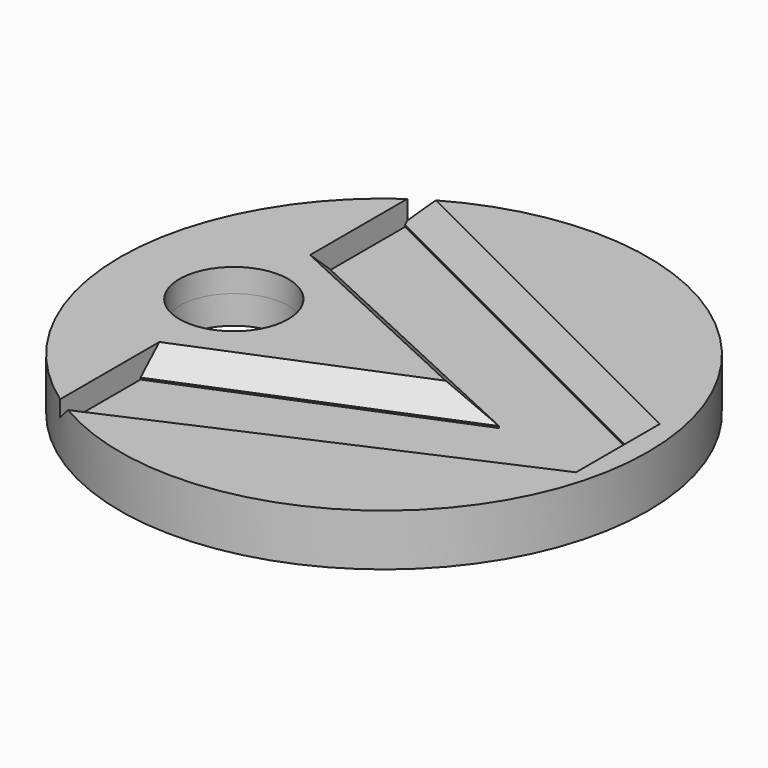
from build123d import *

# Parameters (mm, degrees)
F0_R         = 12.125
F0_R_2       = 2.5
F1_DEPTH     = 2.38
F2_R         = 12.125
F3_DEPTH     = 1.3
F4_T4_DEPTH  = 25.2617303144
F4_T10_DEPTH = 18.811479046
F4_T15_DEPTH = 18.5490461255
F4_T20_DEPTH = 24.8150280867
F5_R         = 2.5
F6_DEPTH     = 25


# Not quite as in the source:
# - a fillet or chamfer that OpenCascade refuses, or shapes differently, is made with other operations: its cross-section is extruded or revolved along the edge and cut away or added


with BuildPart() as f1:
    # F0 (on Top) → F1 (new body)
    with BuildSketch(Plane.XY):
        Circle(F0_R)
        with Locations((-6.9000022486, 0)):
            Circle(F0_R_2, mode=Mode.SUBTRACT)
        Polygon((-6.9049564988, -9.6863286317), (-6.9049564988, -5.3536104666), (5.4957817031, -0.2610715792), (-6.9049564988, 5.4868851832), (-6.9049564988, 9.8370038228), (11.0929343528, 0.8467586343), (11.0929343528, -1.7459120749), align=None, mode=Mode.SUBTRACT)
    extrude(amount=F1_DEPTH)

    # F2 (on Top) → F3 (join)
    with BuildSketch(Plane.XY):
        Circle(F2_R)
    extrude(amount=F3_DEPTH)

    # F4: chamfer of 1 on 4 edges, made by hand


with BuildPart() as f4_tool2:
    # F4_s3 → F4_t4 (new body)
    with BuildSketch(Plane(origin=(-11.7592465012, 5.8739387937, 0), x_dir=(0, 0, 1), z_dir=(0.8946001051, -0.4468676, 0))):
        Polygon((2.38, -6.7145833148), (1.38, -5.7145833148), (2.38, -5.7145833148), align=None)
    extrude(amount=F4_T4_DEPTH)

    split(bisect_by=Plane.YZ.offset(11.0929343528), keep=Keep.BOTTOM)

    split(bisect_by=Plane.YZ.offset(-6.9049564988), keep=Keep.TOP)


with BuildPart() as f1_1:
    add(f1.part)

    # F4_t1: cut F4_tool2
    add(f4_tool2.part, mode=Mode.SUBTRACT)


with BuildPart() as f4_tool8:
    # F4_s9 → F4_t10 (new body)
    with BuildSketch(Plane(origin=(6.9566759614, -3.2245396996, 0), x_dir=(0, 0, 1), z_dir=(-0.907275067, 0.4205376948, 0))):
        Polygon((2.38, 1.0743196339), (1.38, 2.0743196339), (2.38, 2.0743196339), align=None)
    extrude(amount=F4_T10_DEPTH)

    split(bisect_by=Plane.YZ.offset(-6.9049564988), keep=Keep.TOP)


with BuildPart() as f1_2:
    add(f1_1.part)

    # F4_t7: cut F4_tool8
    add(f4_tool8.part, mode=Mode.SUBTRACT)


with BuildPart() as f4_tool13:
    # F4_s14 → F4_t15 (new body)
    with BuildSketch(Plane(origin=(-10.1686835399, -4.1759140075, 0), x_dir=(0, 0, 1), z_dir=(0.9250361088, 0.3798791878, 0))):
        Polygon((2.38, 1.3292337276), (1.38, 2.3292337276), (2.38, 2.3292337276), align=None)
    extrude(amount=F4_T15_DEPTH)

    split(bisect_by=Plane.YZ.offset(-6.9049564988), keep=Keep.TOP)


with BuildPart() as f1_3:
    add(f1_2.part)

    # F4_t12: cut F4_tool13
    add(f4_tool13.part, mode=Mode.SUBTRACT)


with BuildPart() as f4_tool18:
    # F4_s19 → F4_t20 (new body)
    with BuildSketch(Plane(origin=(10.9936482118, 4.8502431202, 0), x_dir=(0, 0, 1), z_dir=(-0.914914599, -0.4036474657, 0))):
        Polygon((2.38, -7.0749952843), (1.38, -6.0749952843), (2.38, -6.0749952843), align=None)
    extrude(amount=F4_T20_DEPTH)

    split(bisect_by=Plane.YZ.offset(11.0929343528), keep=Keep.BOTTOM)

    split(bisect_by=Plane.YZ.offset(-6.9049564988), keep=Keep.TOP)


with BuildPart() as f1_4:
    add(f1_3.part)

    # F4_t17: cut F4_tool18
    add(f4_tool18.part, mode=Mode.SUBTRACT)

    # F5 (on face) → F6 (cut)
    with BuildSketch(Plane.XY.offset(2.38)):
        with Locations((-6.9000022486, 0)):
            Circle(F5_R)
    extrude(amount=-F6_DEPTH, mode=Mode.SUBTRACT)


solid = f1_4.part
